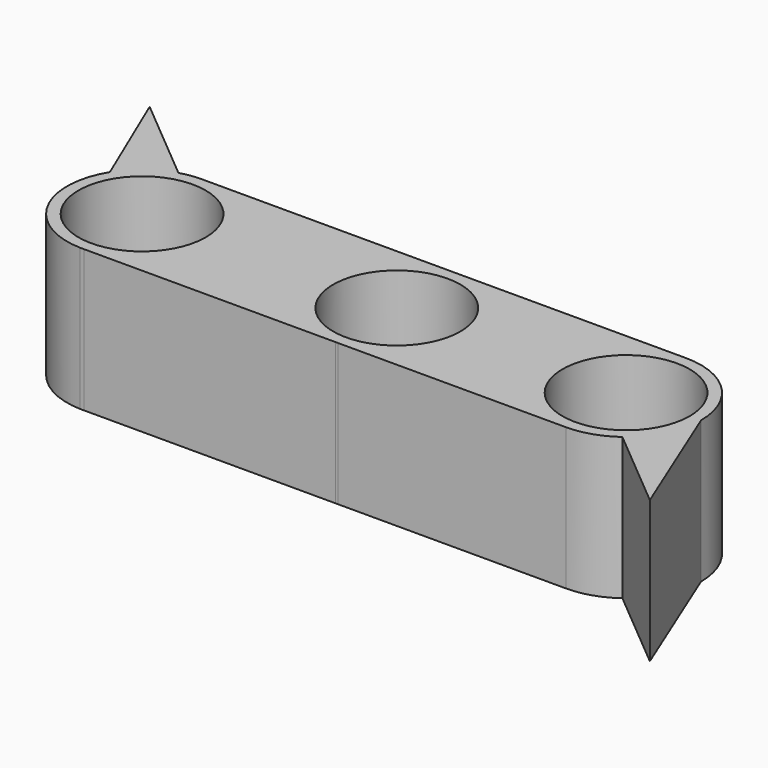
from build123d import *

# Parameters (mm, degrees)
F0_R     = 11.2
F1_DEPTH = 25


# Not quite as in the source:
# - ends of sketch curves that miss each other by under 0.0002 mm in the source are joined


with BuildPart() as f1:
    # F0 (on Top) → F1 (new body)
    with BuildSketch(Plane.XY):
        with BuildLine():
            ThreePointArc((0.2302689957, -13.1979913695), (9.4148699073, -9.2520389444), (13.2, 0))
            ThreePointArc((13.2, 0), (9.3338018159, 9.3338172074), (-2.1767e-05, 13.2))
            ThreePointArc((-2.1767e-05, 13.2), (-13.1994921512, 0.115788384), (-0.2315896221, -13.1979682621))
            Line((-0.2315896221, -13.1979682621), (0.2302689957, -13.1979913695))
        make_face()
        Circle(F0_R, mode=Mode.SUBTRACT)
        with BuildLine():
            ThreePointArc((-2.1767e-05, 13.2), (9.3338018159, 9.3338172074), (13.2, 0))
            ThreePointArc((13.2, 0), (9.4148699073, -9.2520389444), (0.2302689957, -13.1979913695))
            Line((0.2302689957, -13.1979913695), (40.3773476235, -13.1999999835))
            ThreePointArc((40.3773476235, -13.1999999835), (27.1780080417, 0.0003193237), (40.3779862708, 13.2))
            Line((40.3779862708, 13.2), (-2.1767e-05, 13.2))
        make_face()
        with BuildLine():
            ThreePointArc((-0.2315896221, -13.1979682621), (-13.1994921512, 0.115788384), (-2.1767e-05, 13.2))
            Line((-2.1767e-05, 13.2), (-44.8087825295, 13.1998595259))
            ThreePointArc((-44.8087825295, 13.1998595259), (-35.5143647291, 9.3122541296), (-31.6696799576, 0))
            ThreePointArc((-31.6696799576, 0), (-35.4182181161, -9.2146551242), (-44.534811633, -13.1957517105))
            Line((-44.534811633, -13.1957517105), (-0.2315896221, -13.1979682621))
        make_face()
        with BuildLine():
            ThreePointArc((-0.2315896221, -13.1979682621), (-0.0006604143, -13.1999999835), (0.2302689957, -13.1979913695))
            Line((0.2302689957, -13.1979913695), (-0.2315896221, -13.1979682621))
        make_face()
        with BuildLine():
            ThreePointArc((-31.6696799576, 0), (-35.5143647291, 9.3122541296), (-44.8087825295, 13.1998595259))
            ThreePointArc((-44.8087825295, 13.1998595259), (-46.7206749928, 13.0695760214), (-48.593555626, 12.6638363068))
            ThreePointArc((-48.593555626, 12.6638363068), (-52.8729419323, 10.4970375709), (-56.0955079711, 6.9441187643))
            ThreePointArc((-56.0955079711, 6.9441187643), (-56.4810242111, -6.2782708311), (-45.2058686841, -13.1957181366))
            Line((-45.2058686841, -13.1957181366), (-44.534811633, -13.1957517105))
            ThreePointArc((-44.534811633, -13.1957517105), (-35.4182181161, -9.2146551242), (-31.6696799576, 0))
        make_face()
        with Locations((-44.8696799576, 0)):
            Circle(F0_R, mode=Mode.SUBTRACT)
        with BuildLine():
            ThreePointArc((53.5780080378, 0), (49.7118098537, 9.3338172074), (40.3779862708, 13.2))
            ThreePointArc((40.3779862708, 13.2), (27.1780080417, 0.0003193237), (40.3773476235, -13.1999999835))
            ThreePointArc((40.3773476235, -13.1999999835), (44.5067810862, -12.5376725558), (48.2217520277, -10.6167641125))
            ThreePointArc((48.2217520277, -10.6167641125), (52.1631134821, -5.9456950533), (53.5780080378, 0))
        make_face()
        with Locations((40.3780080378, 0)):
            Circle(F0_R, mode=Mode.SUBTRACT)
        with BuildLine():
            ThreePointArc((-45.2058686841, -13.1957181366), (-44.8703403719, -13.1999999835), (-44.534811633, -13.1957517105))
            Line((-44.534811633, -13.1957517105), (-45.2058686841, -13.1957181366))
        make_face()
        with BuildLine():
            ThreePointArc((-56.0955079711, 6.9441187643), (-52.8729419323, 10.4970375709), (-48.593555626, 12.6638363068))
            Line((-48.593555626, 12.6638363068), (-63.987724483, 25.5667958409))
            Line((-63.987724483, 25.5667958409), (-56.0955079711, 6.9441187643))
        make_face()
        with BuildLine():
            Line((62.9060839376, -22.9247582743), (53.5780080378, 0))
            ThreePointArc((53.5780080378, 0), (52.1631134821, -5.9456950533), (48.2217520277, -10.6167641125))
            Line((48.2217520277, -10.6167641125), (62.9060839376, -22.9247582743))
        make_face()
    extrude(amount=F1_DEPTH)


solid = f1.part
